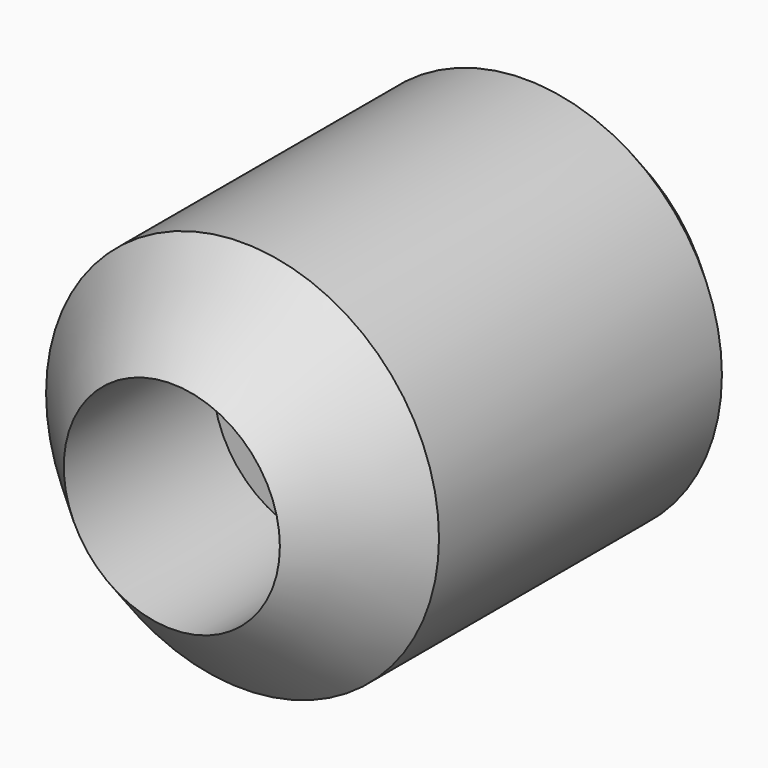
from build123d import *

# Parameters (mm, degrees)
F0_R     = 10
F1_DEPTH = 25
F2_R     = 5.5
F3_DEPTH = 10
F4_SIZE  = 2


# Not quite as in the source:
# - a fillet or chamfer that OpenCascade refuses, or shapes differently, is made with other operations: its cross-section is extruded or revolved along the edge and cut away or added


with BuildPart() as f1:
    # F0 (on Front) → F1 (new body)
    with BuildSketch(Plane.XZ):
        Circle(F0_R)
    extrude(amount=F1_DEPTH)

    # F2 (on face) → F3 (cut)
    with BuildSketch(Plane.XZ.offset(25)):
        Circle(F2_R)
    extrude(amount=-F3_DEPTH, mode=Mode.SUBTRACT)

    # F4
    f4_edges = [f1.edges().sort_by_distance(p)[0] for p in [
        (-10, 0, 0),
    ]]
    chamfer(f4_edges, length=F4_SIZE)

    # F5: chamfer of 5 on 1 edges, made by hand

    # F5_s1 → F5_t2 (revolve, cut)
    with BuildSketch(Plane.XY):
        Polygon((10, -20), (5, -25), (10, -25), align=None)
    revolve(axis=Axis((0, -25, 0), (0, -1, 0)), mode=Mode.SUBTRACT)


solid = f1.part
